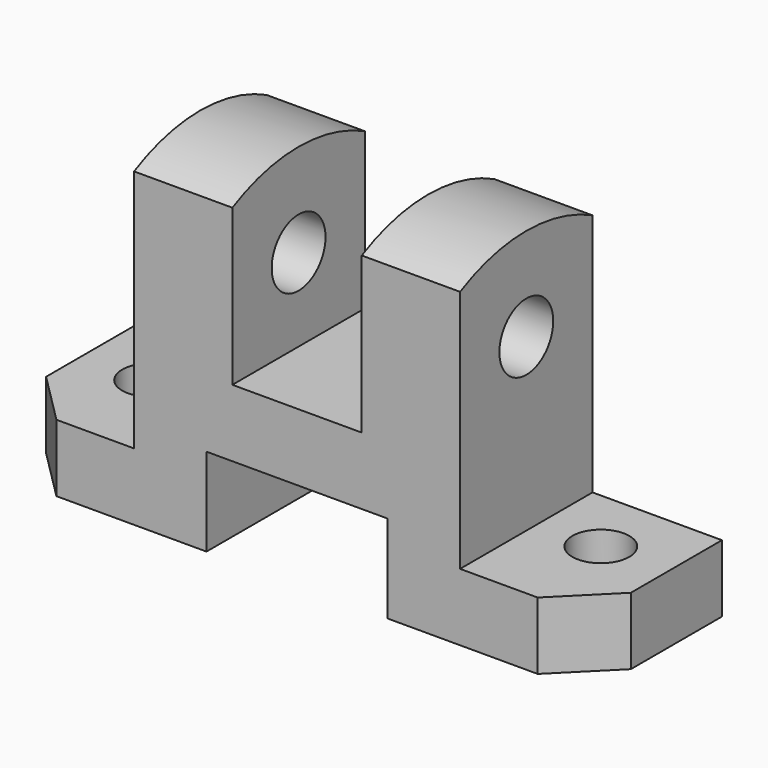
from build123d import *

# Parameters (mm, degrees)
F0_R     = 6.5
F1_DEPTH = 113
F2_W     = 25
F2_H     = 53.8765753508
F2_H_2   = 36.8765753508
F2_W_2   = 35
F2_H_3   = 17
F3_DEPTH = 32.001
F4_R     = 5.5
F5_DEPTH = 64.001


with BuildPart() as f1:
    # F0 (on Right) → F1 (new body)
    with BuildSketch(Plane.YZ):
        with BuildLine():
            Line((0, 60.1287648325), (0, 0))
            Line((0, 0), (32, 0))
            Line((32, 0), (32, 60.1287648325))
            ThreePointArc((32, 60.1287648325), (16, 64), (0, 60.1287648325))
        make_face()
        with Locations((16, 46)):
            Circle(F0_R, mode=Mode.SUBTRACT)
    extrude(amount=F1_DEPTH)

    # F2 (on face) → F3 (cut, through all)
    with BuildSketch(Plane.XZ):
        with Locations((12.5, 39.9382876754)):
            Rectangle(F2_W, F2_H)
        with Locations((100.5, 39.9382876754)):
            Rectangle(F2_W, F2_H)
        with Locations((56.5, 48.4382876754)):
            Rectangle(F2_W, F2_H_2)
        with Locations((56.5, 8.5)):
            Rectangle(F2_W_2, F2_H_3)
    extrude(amount=-F3_DEPTH, mode=Mode.SUBTRACT)

    # F4 (on face) → F5 (cut, through all)
    with BuildSketch(Plane(origin=(0, 0, 0), x_dir=(1, 0, 0), z_dir=(0, 0, -1))):
        Polygon((0, 0), (0, -10), (10, 0), align=None)
        with Locations((100, -19)):
            Circle(F4_R)
        with Locations((13, -19)):
            Circle(F4_R)
        Polygon((113, 0), (103, 0), (113, -10), align=None)
    extrude(amount=-F5_DEPTH, mode=Mode.SUBTRACT)


solid = f1.part
